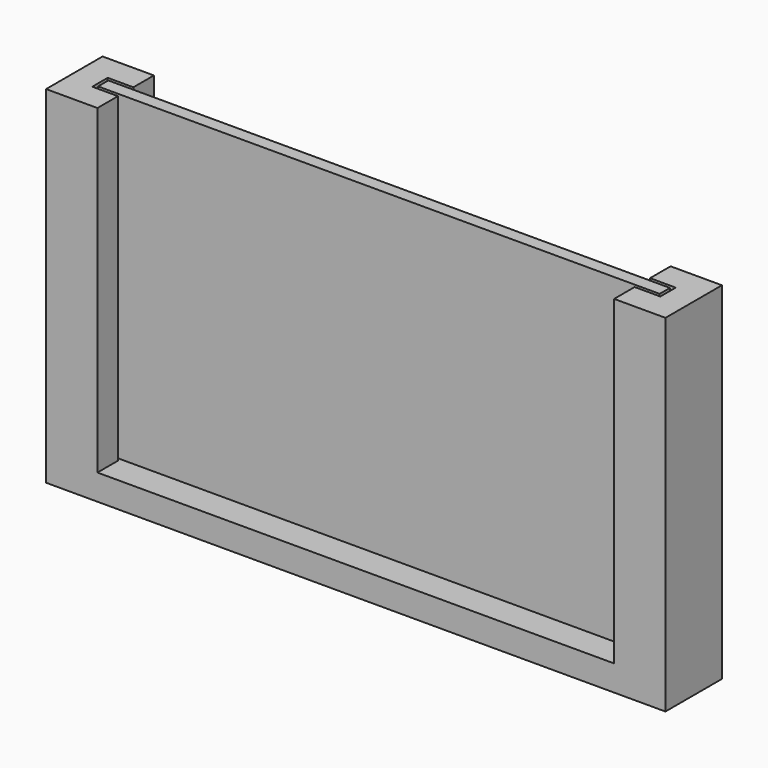
from build123d import *

# Parameters (mm, degrees)
F2_DEPTH = 20
F1_W     = 35
F1_H     = 0.8
F1_W_2   = 32.2
F1_H_2   = 1.6
F3_DEPTH = 1.6
F4_DEPTH = 20


with BuildPart() as f2:
    # F1 (on Top) → F2 (new body)
    with BuildSketch(Plane.XY):
        Polygon((-17.7, -0.6), (-17.7, 0.6), (-16.1, 0.6), (-16.1, 2.2), (-19.3, 2.2), (-19.3, -2.2), (-16.1, -2.2), (-16.1, -0.6), align=None)
    extrude(amount=F2_DEPTH)



with BuildPart() as f2b:
    # F1 (on Top) → F2, piece 2 (new body)
    with BuildSketch(Plane.XY):
        Polygon((16.1, 2.2), (16.1, 0.6), (17.7, 0.6), (17.7, -0.6), (16.1, -0.6), (16.1, -2.2), (19.3, -2.2), (19.3, 2.2), align=None)
    extrude(amount=F2_DEPTH)


with BuildPart() as f2_1:
    add(f2.part)

    add(f2b.part)  # F3 merges F2b
    # F1 (on Top) → F3 (join)
    with BuildSketch(Plane.XY):
        Polygon((-16.1, 0.6), (-17.7, 0.6), (-17.7, -0.6), (-16.1, -0.6), (16.1, -0.6), (17.7, -0.6), (17.7, 0.6), (16.1, 0.6), align=None)
        Rectangle(F1_W, F1_H, mode=Mode.SUBTRACT)
        Rectangle(F1_W, F1_H)
        with Locations((0, 1.4)):
            Rectangle(F1_W_2, F1_H_2)
        with Locations((0, -1.4)):
            Rectangle(F1_W_2, F1_H_2)
        Polygon((-17.7, -0.6), (-17.7, 0.6), (-16.1, 0.6), (-16.1, 2.2), (-19.3, 2.2), (-19.3, -2.2), (-16.1, -2.2), (-16.1, -0.6), align=None)
        Polygon((16.1, 2.2), (16.1, 0.6), (17.7, 0.6), (17.7, -0.6), (16.1, -0.6), (16.1, -2.2), (19.3, -2.2), (19.3, 2.2), align=None)
    extrude(amount=-F3_DEPTH)


with BuildPart() as f4:
    # F1 (on Top) → F4 (new body)
    with BuildSketch(Plane.XY):
        Rectangle(F1_W, F1_H)
    extrude(amount=F4_DEPTH)


solid = Compound([f2_1.part, f4.part])
